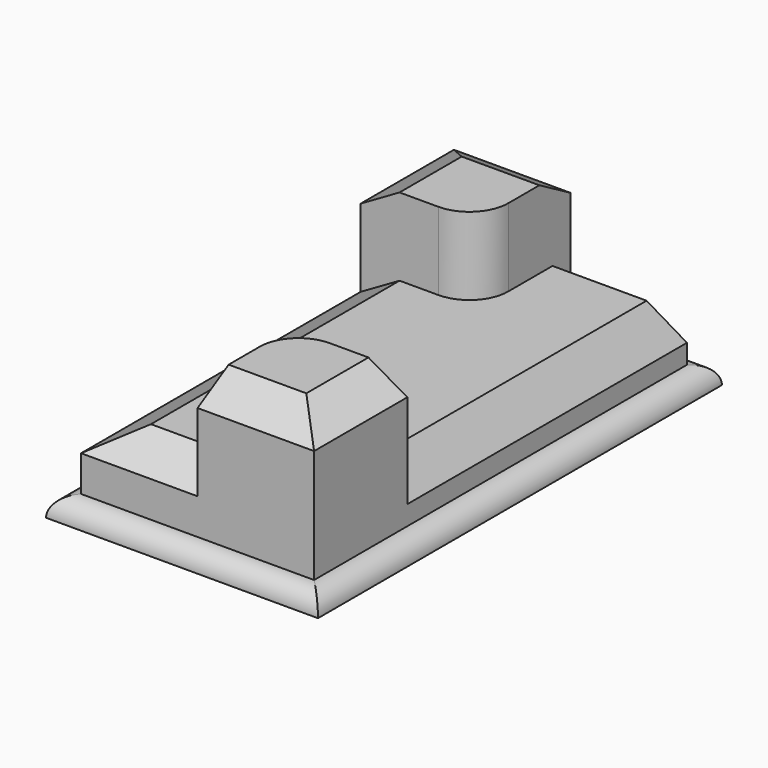
from build123d import *

# Parameters (mm, degrees)
F0_W        = 88.9
F0_H        = 165.1
F1_DEPTH    = 6.35
F2_DEPTH    = 50.8
F3_DEPTH    = 25.4
F4_R        = 6.34999
F5_C1_SIZE2 = 12.7
F5_C1_SIZE  = 7.3323484187
F5_C2_SIZE2 = 12.7
F5_C2_SIZE  = 7.3323484187
F5_C3_SIZE2 = 7.3323484187
F5_C3_SIZE  = 12.7
F5_C4_SIZE2 = 12.7
F5_C4_SIZE  = 7.3323484187
F5_C5_SIZE2 = 7.3323484187
F5_C5_SIZE  = 12.7
F5_C6_SIZE2 = 7.3323484187
F5_C6_SIZE  = 12.7
F6_SIZE2    = 7.3323484187
F6_SIZE     = 12.7


# Not quite as in the source:
# - a fillet or chamfer is up to 0.001 mm smaller than in the source, because OpenCascade refuses the exact size


with BuildPart() as f1:
    # F0 (on Top) → F1 (new body)
    with BuildSketch(Plane.XY):
        with Locations((0, -32.9789540072)):
            Rectangle(F0_W, F0_H)
        Polygon((-38.1, 5.1210459928), (-38.1, 43.2210459928), (0, 43.2210459928), (38.1, 43.2210459928), (38.1, -71.0789540072), (38.1, -109.1789540072), (0, -109.1789540072), (-38.1, -109.1789540072), align=None, mode=Mode.SUBTRACT)
    extrude(amount=F1_DEPTH)

    # F0 (on Top) → F2 (join)
    with BuildSketch(Plane.XY):
        with BuildLine():
            Line((0, 43.2210459928), (-38.1, 43.2210459928))
            Line((-38.1, 43.2210459928), (-38.1, 5.1210459928))
            Line((-38.1, 5.1210459928), (-12.7, 5.1210459928))
            ThreePointArc((-12.7, 5.1210459928), (-3.7197438789, 8.8407898717), (0, 17.8210459928))
            Line((0, 17.8210459928), (0, 43.2210459928))
        make_face()
        with BuildLine():
            Line((38.1, -109.1789540072), (38.1, -71.0789540072))
            Line((38.1, -71.0789540072), (12.7, -71.0789540072))
            ThreePointArc((12.7, -71.0789540072), (3.7197438789, -74.7986978861), (0, -83.7789540072))
            Line((0, -83.7789540072), (0, -109.1789540072))
            Line((0, -109.1789540072), (38.1, -109.1789540072))
        make_face()
    extrude(amount=F2_DEPTH)

    # F0 (on Top) → F3 (join)
    with BuildSketch(Plane.XY):
        with BuildLine():
            Line((38.1, 43.2210459928), (0, 43.2210459928))
            Line((0, 43.2210459928), (0, 17.8210459928))
            ThreePointArc((0, 17.8210459928), (-3.7197438789, 8.8407898717), (-12.7, 5.1210459928))
            Line((-12.7, 5.1210459928), (-38.1, 5.1210459928))
            Line((-38.1, 5.1210459928), (-38.1, -109.1789540072))
            Line((-38.1, -109.1789540072), (0, -109.1789540072))
            Line((0, -109.1789540072), (0, -83.7789540072))
            ThreePointArc((0, -83.7789540072), (3.7197438789, -74.7986978861), (12.7, -71.0789540072))
            Line((12.7, -71.0789540072), (38.1, -71.0789540072))
            Line((38.1, -71.0789540072), (38.1, 43.2210459928))
        make_face()
    extrude(amount=F3_DEPTH)

    # F4 (radius 6.35 in the source; OpenCascade refuses exactly that, so slightly less here)
    f4_edges = [f1.edges().sort_by_distance(p)[0] for p in [
        (44.45, -32.978954, 6.35),
        (0, 49.571046, 6.35),
        (0, -115.528954, 6.35),
        (-44.45, -32.978954, 6.35),
    ]]
    fillet(f4_edges, radius=F4_R)

    # F5: chamfer of 12.7 x 7.3323484187 on 6 edges, made by hand

    # F5_c1
    f5_c1_edges = [f1.edges().sort_by_distance(p)[0] for p in [
        (-38.1, 24.1710459928, 50.8),
    ]]
    f5_c1_side = f1.faces().sort_by_distance((-38.1, 24.1710459928, 50.6533530316))[0]
    chamfer(f5_c1_edges, length=F5_C1_SIZE, length2=F5_C1_SIZE2, reference=f5_c1_side)

    # F5_c2
    f5_c2_edges = [f1.edges().sort_by_distance(p)[0] for p in [
        (-38.1, -52.0289540072, 25.4),
    ]]
    f5_c2_side = f1.faces().sort_by_distance((-38.1, -52.0289540072, 25.2533530316))[0]
    chamfer(f5_c2_edges, length=F5_C2_SIZE, length2=F5_C2_SIZE2, reference=f5_c2_side)

    # F5_c3
    f5_c3_edges = [f1.edges().sort_by_distance(p)[0] for p in [
        (19.05, 43.2210459928, 25.4),
    ]]
    f5_c3_side = f1.faces().sort_by_distance((19.05, 43.2210459928, 25.2533530316))[0]
    chamfer(f5_c3_edges, length=F5_C3_SIZE, length2=F5_C3_SIZE2, reference=f5_c3_side)

    # F5_c4
    f5_c4_edges = [f1.edges().sort_by_distance(p)[0] for p in [
        (-12.7, 43.2210459928, 50.8),
    ]]
    f5_c4_side = f1.faces().sort_by_distance((-12.7, 43.2210459928, 50.6533530316))[0]
    chamfer(f5_c4_edges, length=F5_C4_SIZE, length2=F5_C4_SIZE2, reference=f5_c4_side)

    # F5_c5
    f5_c5_edges = [f1.edges().sort_by_distance(p)[0] for p in [
        (38.1, -17.5951282165, 25.4),
    ]]
    f5_c5_side = f1.faces().sort_by_distance((38.1, -17.5951282165, 25.2533530316))[0]
    chamfer(f5_c5_edges, length=F5_C5_SIZE, length2=F5_C5_SIZE2, reference=f5_c5_side)

    # F5_c6
    f5_c6_edges = [f1.edges().sort_by_distance(p)[0] for p in [
        (-12.7, -109.1789540072, 25.4),
    ]]
    f5_c6_side = f1.faces().sort_by_distance((-12.7, -109.0323070388, 25.4))[0]
    chamfer(f5_c6_edges, length=F5_C6_SIZE, length2=F5_C6_SIZE2, reference=f5_c6_side)

    # F6
    f6_edges = [f1.edges().sort_by_distance(p)[0] for p in [
        (19.05, -109.178954, 50.8),
        (38.1, -90.128954, 50.8),
    ]]
    f6_side = f1.faces().sort_by_distance((19.446042, -90.524996, 50.8))[0]
    chamfer(f6_edges, length=F6_SIZE, length2=F6_SIZE2, reference=f6_side)


solid = f1.part
